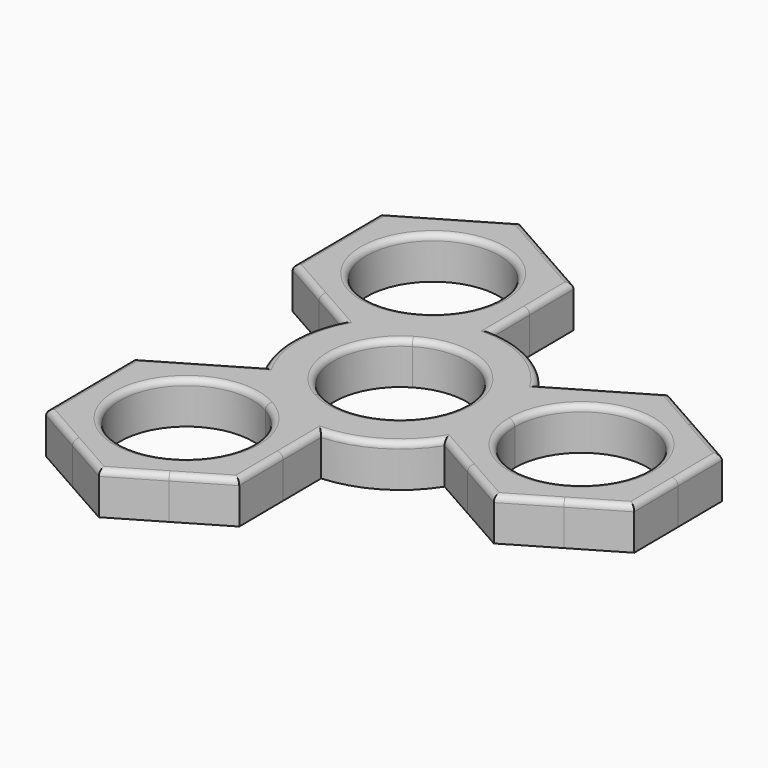
from build123d import *

# Parameters (mm, degrees)
F1_DEPTH = 7
F2_R     = 1


# Not quite as in the source:
# - a feature names something its author has since deleted; it is built from what else it names


with BuildPart() as f1:
    # F0 (on Top) → F1 (new body)
    with BuildSketch(Plane.XY):
        with BuildLine():
            ThreePointArc((11.0496074326, 0.0931428257), (11.0499018577, 0.0465718265), (11.05, 0))
            ThreePointArc((11.05, 0), (5.5652833137, -9.5462098049), (-5.4441396631, -9.6158121513))
            Line((-5.4441396631, -9.6158121513), (-6.8975525143, -12.1829294224))
            Line((-6.897552513, -12.1829294232), (1.1410961503, -16.7341337663))
            Line((1.1410961503, -16.7341337663), (1.1514560176, -17.9631330519))
            ThreePointArc((1.1514560176, -17.9631330519), (9.1310787195, -15.5120405304), (15.1468929184, -9.7247948523))
            Line((15.1468929184, -9.7247948523), (14.0773683822, -9.1192671177))
            Line((14.0773683822, -9.1192671177), (13.9995026293, 0.118009033))
            Line((13.9995026295, 0.1180090099), (11.0496074326, 0.0931428257))
        make_face()
        with BuildLine():
            ThreePointArc((-5.6054677695, 9.5226693256), (5.4441396631, 9.6158121513), (11.0496074326, 0.0931428257))
            Line((11.0496074326, 0.0931428257), (13.9995026295, 0.1180090099))
            Line((13.9995026293, 0.118009033), (13.9216368768, 9.3552851375))
            Line((13.9216368768, 9.3552851375), (14.9808015457, 9.9787566885))
            ThreePointArc((14.9808015457, 9.9787566885), (8.8682818041, 15.6637664003), (0.8484729295, 17.9799914819))
            Line((0.8484729295, 17.9799914819), (0.8588327967, 16.7509921963))
            Line((0.8588327967, 16.7509921963), (-7.1019501115, 12.0649204147))
            Line((-7.1019501152, 12.0649204126), (-5.6054677695, 9.5226693256))
        make_face()
        with BuildLine():
            Line((-6.8975525143, -12.1829294224), (-5.4441396631, -9.6158121513))
            ThreePointArc((-5.4441396631, -9.6158121513), (-11.0496074326, -0.0931428257), (-5.6054677695, 9.5226693256))
            Line((-5.6054677695, 9.5226693256), (-7.1019501152, 12.0649204126))
            Line((-7.1019501115, 12.0649204147), (-15.0627330271, 7.3788486288))
            Line((-15.0627330271, 7.3788486288), (-16.1322575633, 7.9843763634))
            ThreePointArc((-16.1322575633, 7.9843763634), (-17.9993605237, -0.1517258698), (-15.9953658479, -8.2551966296))
            Line((-15.9953658479, -8.2551966296), (-14.936201179, -7.6317250786))
            Line((-14.936201179, -7.6317250786), (-6.897552513, -12.1829294232))
        make_face()
        with BuildLine():
            Line((13.9216368768, 9.3552851375), (13.9995026293, 0.118009033))
            ThreePointArc((13.9995026293, 0.118009033), (14.5071922057, 4.2536176051), (16.0654764727, 8.1179101809))
            ThreePointArc((16.0654764727, 8.1179101809), (15.5509977857, 9.0645721283), (14.9808015457, 9.9787566885))
            Line((14.9808015457, 9.9787566885), (13.9216368768, 9.3552851375))
        make_face()
        with BuildLine():
            Line((17.9993605237, 0.1517258698), (13.9995026295, 0.1180090099))
            ThreePointArc((13.9995026293, 0.118009033), (14.5768374462, -4.0084533342), (16.2000438734, -7.8459275105))
            ThreePointArc((16.2000438734, -7.8459275105), (17.5442410739, -4.0248733073), (18, 0))
            ThreePointArc((18, 0), (17.9998401302, 0.0758636087), (17.9993605237, 0.1517258698))
        make_face()
        with BuildLine():
            ThreePointArc((16.0654764727, 8.1179101809), (14.5071922057, 4.2536176051), (13.9995026293, 0.118009033))
            Line((13.9995026295, 0.1180090099), (17.9993605237, 0.1517258698))
            ThreePointArc((17.9993605237, 0.1517258698), (17.4919496631, 4.2463745694), (16.0654764727, 8.1179101809))
        make_face()
        with BuildLine():
            ThreePointArc((16.2000438734, -7.8459275105), (14.5768374462, -4.0084533342), (13.9995026293, 0.118009033))
            Line((13.9995026293, 0.118009033), (14.0773683822, -9.1192671177))
            Line((14.0773683822, -9.1192671177), (15.1468929184, -9.7247948523))
            ThreePointArc((15.1468929184, -9.7247948523), (15.7015969627, -8.8011279289), (16.2000438734, -7.8459275105))
        make_face()
        with BuildLine():
            Line((1.1410961503, -16.7341337663), (-6.897552513, -12.1829294232))
            ThreePointArc((-6.897552513, -12.1829294232), (-3.5698552065, -14.6904057827), (-1.0024217941, -17.9720658397))
            ThreePointArc((-1.0024217941, -17.9720658397), (0.0746508447, -17.9998452008), (1.1514560176, -17.9631330519))
            Line((1.1514560176, -17.9631330519), (1.1410961503, -16.7341337663))
        make_face()
        with BuildLine():
            Line((-8.8682818041, -15.6637664003), (-6.8975525143, -12.1829294224))
            ThreePointArc((-6.897552513, -12.1829294232), (-10.7598411509, -10.6196848654), (-14.894794477, -10.1066857815))
            ThreePointArc((-14.894794477, -10.1066857815), (-12.2020996077, -13.2328668535), (-8.8682818041, -15.6637664003))
        make_face()
        with BuildLine():
            ThreePointArc((-1.0024217941, -17.9720658397), (-3.5698552065, -14.6904057827), (-6.897552513, -12.1829294232))
            Line((-6.8975525143, -12.1829294224), (-8.8682818041, -15.6637664003))
            ThreePointArc((-8.8682818041, -15.6637664003), (-5.0685065805, -17.2716600547), (-1.0024217941, -17.9720658397))
        make_face()
        with BuildLine():
            ThreePointArc((-14.894794477, -10.1066857815), (-10.7598411509, -10.6196848654), (-6.897552513, -12.1829294232))
            Line((-6.897552513, -12.1829294232), (-14.936201179, -7.6317250786))
            Line((-14.936201179, -7.6317250786), (-15.9953658479, -8.2551966296))
            ThreePointArc((-15.9953658479, -8.2551966296), (-15.4727988497, -9.1974178852), (-14.894794477, -10.1066857815))
        make_face()
        with BuildLine():
            Line((-15.0627330271, 7.3788486288), (-7.1019501115, 12.0649204147))
            ThreePointArc((-7.1019501115, 12.0649204147), (-10.9373369937, 10.4367881888), (-15.0630546786, 9.8541556588))
            ThreePointArc((-15.0630546786, 9.8541556588), (-15.6256486304, 8.9352730724), (-16.1322575633, 7.9843763634))
            Line((-16.1322575633, 7.9843763634), (-15.0627330271, 7.3788486288))
        make_face()
        with BuildLine():
            Line((-9.1310787195, 15.5120405304), (-7.1019501152, 12.0649204126))
            ThreePointArc((-7.1019501115, 12.0649204147), (-3.8169962962, 14.6281382121), (-1.3052493964, 17.952613292))
            ThreePointArc((-1.3052493964, 17.952613292), (-5.3589490562, 17.1837616666), (-9.1310787195, 15.5120405304))
        make_face()
        with BuildLine():
            ThreePointArc((-15.0630546786, 9.8541556588), (-10.9373369937, 10.4367881888), (-7.1019501115, 12.0649204147))
            Line((-7.1019501152, 12.0649204126), (-9.1310787195, 15.5120405304))
            ThreePointArc((-9.1310787195, 15.5120405304), (-12.4234430826, 13.0252854853), (-15.0630546786, 9.8541556588))
        make_face()
        with BuildLine():
            ThreePointArc((-1.3052493964, 17.952613292), (-3.8169962962, 14.6281382121), (-7.1019501115, 12.0649204147))
            Line((-7.1019501115, 12.0649204147), (0.8588327967, 16.7509921963))
            Line((0.8588327967, 16.7509921963), (0.8484729295, 17.9799914819))
            ThreePointArc((0.8484729295, 17.9799914819), (-0.2287981129, 17.9985458141), (-1.3052493964, 17.952613292))
        make_face()
        with BuildLine():
            ThreePointArc((21.8824200464, 14.0413570729), (18.5830627592, 11.4634910229), (16.0654764727, 8.1179101809))
            ThreePointArc((16.0654764727, 8.1179101809), (17.4919496631, 4.2463745694), (17.9993605237, 0.1517258698))
            ThreePointArc((17.9993605237, 0.1517258698), (17.9998401302, 0.0758636087), (18, 0))
            ThreePointArc((18, 0), (17.5442410739, -4.0248733073), (16.2000438734, -7.8459275105))
            ThreePointArc((16.2000438734, -7.8459275105), (18.7736715236, -11.1485917762), (22.1160170248, -13.6704714491))
            ThreePointArc((22.1160170248, -13.6704714491), (30.1338017827, -15.7465551257), (38.115448881, -13.5356038702))
            ThreePointArc((38.115448881, -13.5356038702), (43.8889348324, -7.6886525341), (45.9989342061, 0.2528764497))
            ThreePointArc((45.9989342061, 0.2528764497), (45.9987921004, 0.3203105864), (45.9983657857, 0.3877435252))
            ThreePointArc((45.9983657857, 0.3877435252), (43.7874147818, 8.3693906901), (37.8818514056, 14.1762243383))
            ThreePointArc((37.8818514056, 14.1762243383), (29.8640669388, 16.2523080278), (21.8824200464, 14.0413570729))
        make_face()
        with BuildLine():
            ThreePointArc((41.0489342061, 0.2528764497), (30.0455060326, -10.797025408), (18.9493267735, 0.1597336241))
            ThreePointArc((18.9493267735, 0.1597336241), (29.9523623796, 11.3027783075), (41.0489342061, 0.2528764497))
        make_face(mode=Mode.SUBTRACT)
        with BuildLine():
            ThreePointArc((14.9808015457, 9.9787566885), (15.5509977857, 9.0645721283), (16.0654764727, 8.1179101809))
            ThreePointArc((16.0654764727, 8.1179101809), (18.5830627592, 11.4634910229), (21.8824200464, 14.0413570729))
            Line((21.8824200464, 14.0413570729), (14.9808015457, 9.9787566885))
        make_face()
        with BuildLine():
            ThreePointArc((22.1160170248, -13.6704714491), (18.7736715236, -11.1485917762), (16.2000438734, -7.8459275105))
            ThreePointArc((16.2000438734, -7.8459275105), (15.7015969627, -8.8011279289), (15.1468929184, -9.7247948523))
            Line((15.1468929184, -9.7247948523), (22.1160170248, -13.6704714491))
        make_face()
        with BuildLine():
            ThreePointArc((1.2189619052, -25.971410148), (0.6361430563, -21.8251499194), (-1.0024217941, -17.9720658397))
            ThreePointArc((-1.0024217941, -17.9720658397), (-5.0685065805, -17.2716600547), (-8.8682818041, -15.6637664003))
            ThreePointArc((-8.8682818041, -15.6637664003), (-12.2020996077, -13.2328668535), (-14.894794477, -10.1066857815))
            ThreePointArc((-14.894794477, -10.1066857815), (-19.0417996452, -10.6841806257), (-22.8969844066, -12.3177970481))
            ThreePointArc((-22.8969844066, -12.3177970481), (-28.7038176566, -18.2233603011), (-30.7799012508, -26.2411446982))
            ThreePointArc((-30.7799012508, -26.2411446982), (-28.5689501674, -34.2227917132), (-22.6633868436, -40.029625239))
            ThreePointArc((-22.6633868436, -40.029625239), (-14.6456020905, -42.1057089092), (-6.6639549987, -39.8947576537))
            ThreePointArc((-6.6639549987, -39.8947576537), (-0.8904690472, -34.0478063176), (1.2195303265, -26.1062773338))
            ThreePointArc((1.2195303265, -26.1062773338), (1.2193882205, -26.038843142), (1.2189619052, -25.971410148))
        make_face()
        with BuildLine():
            ThreePointArc((-3.7304696735, -26.1062773338), (-24.3266794784, -31.6715606475), (-9.3363300105, -16.4904651825))
            ThreePointArc((-9.3363300105, -16.4904651825), (-5.2342598687, -20.5409940201), (-3.7304696735, -26.1062773338))
        make_face(mode=Mode.SUBTRACT)
        with BuildLine():
            ThreePointArc((1.1514560176, -17.9631330519), (0.0746508447, -17.9998452008), (-1.0024217941, -17.9720658397))
            ThreePointArc((-1.0024217941, -17.9720658397), (0.6361430563, -21.8251499194), (1.2189619052, -25.971410148))
            Line((1.2189619052, -25.971410148), (1.1514560176, -17.9631330519))
        make_face()
        with BuildLine():
            ThreePointArc((-22.8969844066, -12.3177970481), (-19.0417996452, -10.6841806257), (-14.894794477, -10.1066857815))
            ThreePointArc((-14.894794477, -10.1066857815), (-15.4727988497, -9.1974178852), (-15.9953658479, -8.2551966296))
            Line((-15.9953658479, -8.2551966296), (-22.8969844066, -12.3177970481))
        make_face()
        with BuildLine():
            ThreePointArc((-23.1013817149, 11.9300529858), (-19.2192056896, 10.3616588841), (-15.0630546786, 9.8541556588))
            ThreePointArc((-15.0630546786, 9.8541556588), (-12.4234430826, 13.0252854853), (-9.1310787195, 15.5120405304))
            ThreePointArc((-9.1310787195, 15.5120405304), (-5.3589490562, 17.1837616666), (-1.3052493964, 17.952613292))
            ThreePointArc((-1.3052493964, 17.952613292), (0.2510448679, 21.7675375835), (0.7815354675, 25.8534008841))
            ThreePointArc((0.7815354675, 25.8534008841), (0.7813933621, 25.9208349314), (0.7809670486, 25.9882677809))
            ThreePointArc((0.7809670486, 25.9882677809), (-1.4299839201, 33.969915062), (-7.3355473625, 39.7767487893))
            ThreePointArc((-7.3355473625, 39.7767487893), (-15.3533321156, 41.8528324594), (-23.3349792074, 39.641881204))
            ThreePointArc((-23.3349792074, 39.641881204), (-29.1418124989, 33.7363179461), (-31.2178961098, 25.7185335197))
            ThreePointArc((-31.2178961098, 25.7185335197), (-29.0069450299, 17.7368865107), (-23.1013817149, 11.9300529858))
        make_face()
        with BuildLine():
            ThreePointArc((-4.1684645325, 25.8534008841), (-5.6256829012, 20.36878234), (-9.6129967631, 16.3307315584))
            ThreePointArc((-9.6129967631, 16.3307315584), (-24.8112461639, 31.3380194281), (-4.1684645325, 25.8534008841))
        make_face(mode=Mode.SUBTRACT)
        with BuildLine():
            ThreePointArc((-16.1322575633, 7.9843763634), (-15.6256486304, 8.9352730724), (-15.0630546786, 9.8541556588))
            ThreePointArc((-15.0630546786, 9.8541556588), (-19.2192056896, 10.3616588841), (-23.1013817149, 11.9300529858))
            Line((-23.1013817149, 11.9300529858), (-16.1322575633, 7.9843763634))
        make_face()
        with BuildLine():
            ThreePointArc((0.7815354675, 25.8534008841), (0.2510448679, 21.7675375835), (-1.3052493964, 17.952613292))
            ThreePointArc((-1.3052493964, 17.952613292), (-0.2287981129, 17.9985458141), (0.8484729295, 17.9799914819))
            Line((0.8484729295, 17.9799914819), (0.7809670486, 25.9882677809))
            ThreePointArc((0.7809670486, 25.9882677809), (0.7813933621, 25.9208349314), (0.7815354675, 25.8534008841))
        make_face()
        with BuildLine():
            Line((29.8432027007, 18.727428705), (21.8824200464, 14.0413570729))
            ThreePointArc((21.8824200464, 14.0413570729), (29.8640669388, 16.2523080278), (37.8818514056, 14.1762243383))
            Line((37.8818514056, 14.1762243383), (29.8432027007, 18.727428705))
        make_face()
        with BuildLine():
            ThreePointArc((38.115448881, -13.5356038702), (30.1338017827, -15.7465551257), (22.1160170248, -13.6704714491))
            Line((22.1160170248, -13.6704714491), (30.1546657115, -18.2216758055))
            Line((30.1546657115, -18.2216758055), (38.115448881, -13.5356038702))
        make_face()
        with BuildLine():
            Line((1.2968276557, -35.2086860216), (1.2189619052, -25.971410148))
            ThreePointArc((1.2189619052, -25.971410148), (1.2193882205, -26.038843142), (1.2195303265, -26.1062773338))
            ThreePointArc((1.2195303265, -26.1062773338), (-0.8904690472, -34.0478063176), (-6.6639549987, -39.8947576537))
            Line((-6.6639549987, -39.8947576537), (1.2968276557, -35.2086860216))
        make_face()
        with BuildLine():
            ThreePointArc((-30.7799012508, -26.2411446982), (-28.7038176566, -18.2233603011), (-22.8969844066, -12.3177970481))
            Line((-22.8969844066, -12.3177970481), (-30.8577670028, -17.003868646))
            Line((-30.8577670028, -17.003868646), (-30.7799012508, -26.2411446982))
        make_face()
        with BuildLine():
            Line((-31.1400303564, 16.4812573166), (-23.1013817149, 11.9300529858))
            ThreePointArc((-23.1013817149, 11.9300529858), (-29.0069450299, 17.7368865107), (-31.2178961098, 25.7185335197))
            Line((-31.2178961098, 25.7185335197), (-31.1400303564, 16.4812573166))
        make_face()
        with BuildLine():
            Line((45.92050003, 9.6250200172), (37.8818514056, 14.1762243383))
            ThreePointArc((37.8818514056, 14.1762243383), (43.7874147818, 8.3693906901), (45.9983657857, 0.3877435252))
            Line((45.9983657857, 0.3877435252), (45.92050003, 9.6250200172))
        make_face()
        with BuildLine():
            ThreePointArc((45.9989342061, 0.2528764497), (43.8889348324, -7.6886525341), (38.115448881, -13.5356038702))
            Line((38.115448881, -13.5356038702), (46.0762315354, -8.849532238))
            Line((46.0762315354, -8.849532238), (45.9983657857, 0.3877435252))
            ThreePointArc((45.9983657857, 0.3877435252), (45.9987921004, 0.3203105864), (45.9989342061, 0.2528764497))
        make_face()
        with BuildLine():
            ThreePointArc((-22.6633868436, -40.029625239), (-28.5689501674, -34.2227917132), (-30.7799012508, -26.2411446982))
            Line((-30.7799012508, -26.2411446982), (-30.7020354974, -35.4784209013))
            Line((-30.7020354974, -35.4784209013), (-22.6633868436, -40.029625239))
        make_face()
        with BuildLine():
            Line((-31.2957618618, 34.9558095718), (-31.2178961098, 25.7185335197))
            ThreePointArc((-31.2178961098, 25.7185335197), (-29.1418124989, 33.7363179461), (-23.3349792074, 39.641881204))
            Line((-23.3349792074, 39.641881204), (-31.2957618618, 34.9558095718))
        make_face()
        with BuildLine():
            ThreePointArc((-7.3355473625, 39.7767487893), (-1.4299839201, 33.969915062), (0.7809670486, 25.9882677809))
            Line((0.7809670486, 25.9882677809), (0.7031012913, 35.2255444515))
            Line((0.7031012913, 35.2255444515), (-7.3355473625, 39.7767487893))
        make_face()
        with BuildLine():
            Line((-14.6247381681, -44.580829589), (-6.6639549987, -39.8947576537))
            ThreePointArc((-6.6639549987, -39.8947576537), (-14.6456020905, -42.1057089092), (-22.6633868436, -40.029625239))
            Line((-22.6633868436, -40.029625239), (-14.6247381681, -44.580829589))
        make_face()
        with BuildLine():
            Line((-15.374196038, 44.3279531393), (-23.3349792074, 39.641881204))
            ThreePointArc((-23.3349792074, 39.641881204), (-15.3533321156, 41.8528324594), (-7.3355473625, 39.7767487893))
            Line((-7.3355473625, 39.7767487893), (-15.374196038, 44.3279531393))
        make_face()
    extrude(amount=F1_DEPTH)

    # F2 (call 1 of 5: OpenCascade refuses the feature's edges together)
    f2_edges = [f1.edges().sort_by_distance(p)[0] for p in [
        (-11.05, 0, 7),
    ]]
    fillet(f2_edges, radius=F2_R)

    # F2#2 (call 2 of 5)
    f2_2_edges = [f1.edges().sort_by_distance(p)[0] for p in [
        (9.131079, -15.512041, 7),
        (22.650779, -13.973235, 7),
        (38.115449, -13.535604, 7),
        (45.998366, 0.387744, 7),
        (37.881851, 14.176224, 7),
        (22.412002, 14.353093, 7),
        (8.868282, 15.663766, 7),
        (0.775787, 26.602768, 7),
        (-7.335547, 39.776749, 7),
        (-23.334979, 39.641881, 7),
        (-31.217896, 25.718533, 7),
        (-23.636144, 12.232817, 7),
        (-17.999361, -0.151726, 7),
        (-23.426566, -12.629533, 7),
        (-30.779901, -26.241145, 7),
        (-22.663387, -40.029625, 7),
        (-6.663955, -39.894758, 7),
        (1.224142, -26.58591, 7),
    ]]
    fillet(f2_2_edges, radius=F2_R)

    # F2#3 (call 3 of 5)
    f2_3_edges = [f1.edges().sort_by_distance(p)[0] for p in [
        (-25.83047, -26.106277, 7),
    ]]
    fillet(f2_3_edges, radius=F2_R)

    # F2#4 (call 4 of 5)
    f2_4_edges = [f1.edges().sort_by_distance(p)[0] for p in [
        (18.948934, 0.252876, 7),
    ]]
    fillet(f2_4_edges, radius=F2_R)

    # F2#5 (call 5 of 5)
    f2_5_edges = [f1.edges().sort_by_distance(p)[0] for p in [
        (-26.268465, 25.853401, 7),
    ]]
    fillet(f2_5_edges, radius=F2_R)


solid = f1.part
